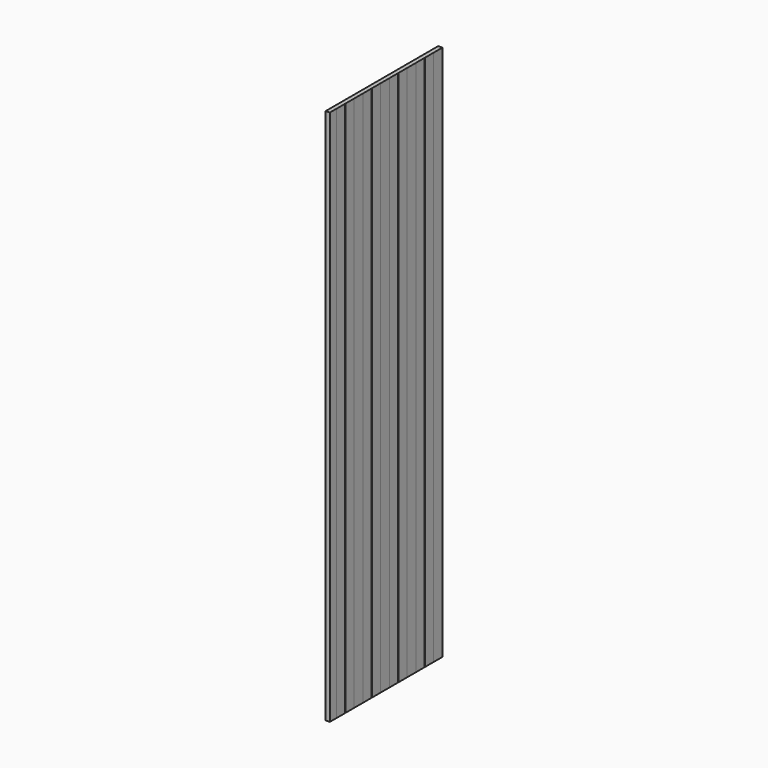
from build123d import *

# Parameters (mm, degrees)
F0_W     = 647.7
F0_H     = 2470.15
F1_DEPTH = 19.05
F3_R     = 4.7625
F4_DEPTH = 34.925
F6_DEPTH = 2540


# Not quite as in the source:
# - ends of sketch curves that miss each other by under 0.0002 mm in the source are joined


with BuildPart() as f1:
    # F0 (on Right) → F1 (new body)
    with BuildSketch(Plane.YZ):
        with Locations((-323.85, 1235.075)):
            Rectangle(F0_W, F0_H)
    extrude(amount=F1_DEPTH)

    # F3 (on offset) → F4 (cut)
    with BuildSketch(Plane.YZ.offset(-25.4)):
        with Locations((-9.525, 76.2)):
            Circle(F3_R)
        with Locations((-295.275, 1384.3)):
            Circle(F3_R)
        with Locations((-295.275, 2114.55)):
            Circle(F3_R)
        with Locations((-295.275, 2406.65)):
            Circle(F3_R)
        with Locations((-9.525, 2444.75)):
            Circle(F3_R)
        with Locations((-9.525, 2114.55)):
            Circle(F3_R)
        with Locations((-9.525, 1384.3)):
            Circle(F3_R)
        with Locations((-9.525, 901.7)):
            Circle(F3_R)
        with Locations((-9.525, 177.8)):
            Circle(F3_R)
        with Locations((-9.525, 514.35)):
            Circle(F3_R)
        with Locations((-9.525, 1612.9)):
            Circle(F3_R)
        with Locations((-9.525, 1841.5)):
            Circle(F3_R)
    extrude(amount=F4_DEPTH, mode=Mode.SUBTRACT)

    # F5 (on Top) → F6 (cut)
    with BuildSketch(Plane.XY):
        with BuildLine():
            ThreePointArc((18.5439819652, 50.8019742476), (18.9026076156, 50.6517855308), (19.0499961487, 50.292))
            ThreePointArc((19.0499961487, 50.292), (19.558, 50.8), (19.0499961487, 51.308))
            ThreePointArc((19.0499961487, 51.308), (18.9012115958, 50.95076922), (18.5439819652, 50.8019742476))
        make_face()
        with BuildLine():
            ThreePointArc((18.5439819652, 0.0019742476), (18.9026076156, -0.1482144692), (19.0499961487, -0.508))
            ThreePointArc((19.0499961487, -0.508), (19.558, 0), (19.0499961487, 0.508))
            ThreePointArc((19.0499961487, 0.508), (18.9012115958, 0.15076922), (18.5439819652, 0.0019742476))
        make_face()
        with BuildLine():
            ThreePointArc((18.5439819652, -50.7980257524), (18.9026076156, -50.9482144692), (19.0499961487, -51.308))
            ThreePointArc((19.0499961487, -51.308), (19.558, -50.8), (19.0499961487, -50.292))
            ThreePointArc((19.0499961487, -50.292), (18.9012115958, -50.64923078), (18.5439819652, -50.7980257524))
        make_face()
        with BuildLine():
            ThreePointArc((18.5439819652, -101.5980257524), (18.9026076156, -101.7482144692), (19.0499961487, -102.108))
            ThreePointArc((19.0499961487, -102.108), (19.558, -101.6), (19.0499961487, -101.092))
            ThreePointArc((19.0499961487, -101.092), (18.9012115958, -101.44923078), (18.5439819652, -101.5980257524))
        make_face()
        with BuildLine():
            ThreePointArc((18.5439819652, -152.3980257524), (18.9026076156, -152.5482144692), (19.0499961487, -152.908))
            ThreePointArc((19.0499961487, -152.908), (19.558, -152.4), (19.0499961487, -151.892))
            ThreePointArc((19.0499961487, -151.892), (18.9012115958, -152.24923078), (18.5439819652, -152.3980257524))
        make_face()
        with BuildLine():
            ThreePointArc((18.5439819652, -203.1980257524), (18.9026076156, -203.3482144692), (19.0499961487, -203.708))
            ThreePointArc((19.0499961487, -203.708), (19.558, -203.2), (19.0499961487, -202.692))
            ThreePointArc((19.0499961487, -202.692), (18.9012115958, -203.04923078), (18.5439819652, -203.1980257524))
        make_face()
        with BuildLine():
            ThreePointArc((18.5439819652, -253.9980257524), (18.9026076156, -254.1482144692), (19.0499961487, -254.508))
            ThreePointArc((19.0499961487, -254.508), (19.558, -254), (19.0499961487, -253.492))
            ThreePointArc((19.0499961487, -253.492), (18.9012115958, -253.84923078), (18.5439819652, -253.9980257524))
        make_face()
        with BuildLine():
            ThreePointArc((18.5439819652, -304.7980257524), (18.9026076156, -304.9482144692), (19.0499961487, -305.308))
            ThreePointArc((19.0499961487, -305.308), (19.558, -304.8), (19.0499961487, -304.292))
            ThreePointArc((19.0499961487, -304.292), (18.9012115958, -304.64923078), (18.5439819652, -304.7980257524))
        make_face()
        with BuildLine():
            ThreePointArc((18.5439819652, -355.5980257524), (18.9026076156, -355.7482144692), (19.0499961487, -356.108))
            ThreePointArc((19.0499961487, -356.108), (19.558, -355.6), (19.0499961487, -355.092))
            ThreePointArc((19.0499961487, -355.092), (18.9012115958, -355.44923078), (18.5439819652, -355.5980257524))
        make_face()
        with BuildLine():
            ThreePointArc((18.5439819652, -406.3980257524), (18.9026076156, -406.5482144692), (19.0499961487, -406.908))
            ThreePointArc((19.0499961487, -406.908), (19.558, -406.4), (19.0499961487, -405.892))
            ThreePointArc((19.0499961487, -405.892), (18.9012115958, -406.24923078), (18.5439819652, -406.3980257524))
        make_face()
        with BuildLine():
            ThreePointArc((18.5439819652, -457.1980257524), (18.9026076156, -457.3482144692), (19.0499961487, -457.708))
            ThreePointArc((19.0499961487, -457.708), (19.558, -457.2), (19.0499961487, -456.692))
            ThreePointArc((19.0499961487, -456.692), (18.9012115958, -457.04923078), (18.5439819652, -457.1980257524))
        make_face()
        with BuildLine():
            ThreePointArc((18.5439819652, -507.9980257524), (18.9026076156, -508.1482144692), (19.0499961487, -508.508))
            ThreePointArc((19.0499961487, -508.508), (19.558, -508), (19.0499961487, -507.492))
            ThreePointArc((19.0499961487, -507.492), (18.9012115958, -507.84923078), (18.5439819652, -507.9980257524))
        make_face()
        with BuildLine():
            ThreePointArc((18.5439819652, -558.7980257524), (18.9026076156, -558.9482144692), (19.0499961487, -559.308))
            ThreePointArc((19.0499961487, -559.308), (19.558, -558.8), (19.0499961487, -558.292))
            ThreePointArc((19.0499961487, -558.292), (18.9012115958, -558.64923078), (18.5439819652, -558.7980257524))
        make_face()
        with BuildLine():
            ThreePointArc((18.5439819652, -609.5980257524), (18.9026076156, -609.7482144692), (19.0499961487, -610.108))
            ThreePointArc((19.0499961487, -610.108), (19.558, -609.6), (19.0499961487, -609.092))
            ThreePointArc((19.0499961487, -609.092), (18.9012115958, -609.44923078), (18.5439819652, -609.5980257524))
        make_face()
        with BuildLine():
            ThreePointArc((18.5439819652, -660.3980257524), (18.9026076156, -660.5482144692), (19.0499961487, -660.908))
            ThreePointArc((19.0499961487, -660.908), (19.558, -660.4), (19.0499961487, -659.892))
            ThreePointArc((19.0499961487, -659.892), (18.9012115958, -660.24923078), (18.5439819652, -660.3980257524))
        make_face()
        with BuildLine():
            ThreePointArc((18.5439819652, -711.1980257524), (18.9026076156, -711.3482144692), (19.0499961487, -711.708))
            ThreePointArc((19.0499961487, -711.708), (19.558, -711.2), (19.0499961487, -710.692))
            ThreePointArc((19.0499961487, -710.692), (18.9012115958, -711.04923078), (18.5439819652, -711.1980257524))
        make_face()
    extrude(amount=F6_DEPTH, mode=Mode.SUBTRACT)


solid = f1.part
